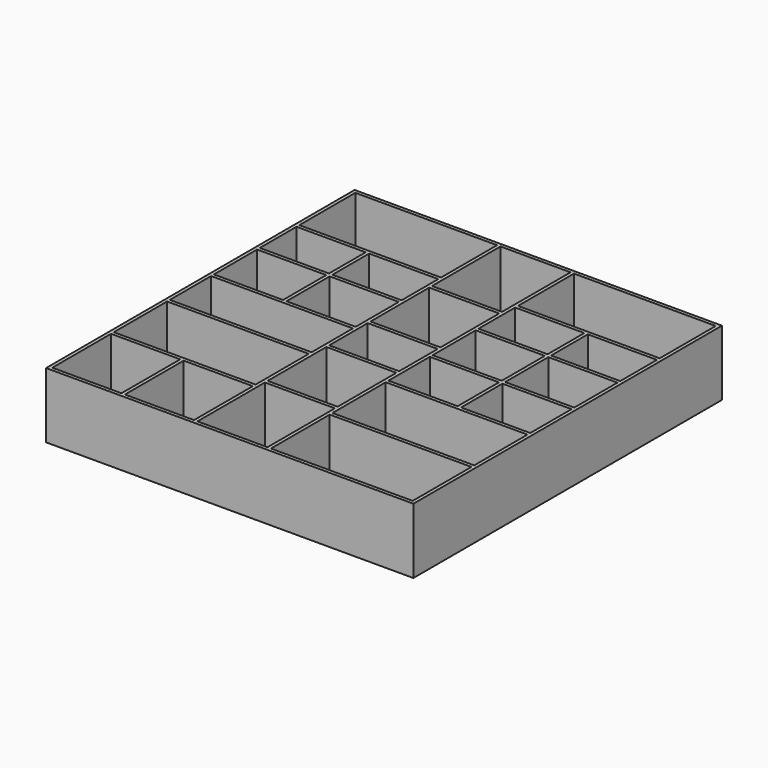
from build123d import *

# Parameters (mm, degrees)
F0_W     = 784.225
F0_H     = 387.35
F0_W_2   = 382.5875
F0_H_2   = 406.4
F0_H_3   = 254
F0_W_3   = 387.35
F0_H_4   = 473.7870542765
F0_W_4   = 19.05
F0_H_5   = 19.05
F0_H_6   = 368.3
F0_H_7   = 298.45
F0_H_8   = 466.0129457235
F0_H_9   = 285.75
F0_H_10  = 266.7
F1_DEPTH = 6.35
F2_DEPTH = 355.6


with BuildPart() as f1:
    # F0 (on Top) → F1 (new body)
    with BuildSketch(Plane.XY):
        Polygon((-1882.2203393722, 1059.8308014154), (-1901.2703393722, 1059.8308014154), (-1901.2703393722, -1073.7691985846), (-1882.2203393722, -1073.7691985846), (-1882.2203393722, -1054.7191985846), (-1882.2203393722, -648.3191985846), (-1882.2203393722, -629.2691985846), (-1882.2203393722, -260.9691985846), (-1882.2203393722, -241.9191985846), (-1882.2203393722, 43.8308014154), (-1882.2203393722, 62.8808014154), (-1882.2203393722, 361.3308014154), (-1882.2203393722, 380.3808014154), (-1882.2203393722, 634.3808014154), (-1882.2203393722, 653.4308014154), (-1882.2203393722, 1040.7808014154), align=None)
        Polygon((-682.0703393722, 1059.8308014154), (-1882.2203393722, 1059.8308014154), (-1882.2203393722, 1040.7808014154), (-1097.9953393722, 1040.7808014154), (-1078.9453393722, 1040.7808014154), (-691.5953393722, 1040.7808014154), (-672.5453393722, 1040.7808014154), (111.6796606278, 1040.7808014154), (111.6796606278, 1059.8308014154), align=None)
        with Locations((-1490.1078393722, 847.1058014154)):
            Rectangle(F0_W, F0_H)
        Polygon((-1882.2203393722, -1054.7191985846), (-1882.2203393722, -1073.7691985846), (111.6796606278, -1073.7691985846), (111.6796606278, -1054.7191985846), (-672.5453393722, -1054.7191985846), (-691.5953393722, -1054.7191985846), (-1078.9453393722, -1054.7191985846), (-1097.9953393722, -1054.7191985846), (-1480.5828393722, -1054.7191985846), (-1499.6328393722, -1054.7191985846), align=None)
        Polygon((130.7296606278, 1059.8308014154), (111.6796606278, 1059.8308014154), (111.6796606278, 1040.7808014154), (111.6796606278, 653.4308014154), (111.6796606278, 634.3808014154), (111.6796606278, 380.3808014154), (111.6796606278, 361.3308014154), (111.6796606278, 62.8808014154), (111.6796606278, 43.8308014154), (111.6796606278, -241.9191985846), (111.6796606278, -260.9691985846), (111.6796606278, -629.2691985846), (111.6796606278, -648.3191985846), (111.6796606278, -1054.7191985846), (111.6796606278, -1073.7691985846), (130.7296606278, -1073.7691985846), align=None)
        Polygon((-1097.9953393722, 653.4308014154), (-1882.2203393722, 653.4308014154), (-1882.2203393722, 634.3808014154), (-1499.6328393722, 634.3808014154), (-1480.5828393722, 634.3808014154), (-1097.9953393722, 634.3808014154), align=None)
        Polygon((-1078.9453393722, 1040.7808014154), (-1097.9953393722, 1040.7808014154), (-1097.9953393722, 653.4308014154), (-1097.9953393722, 634.3808014154), (-1097.9953393722, 380.3808014154), (-1097.9953393722, 361.3308014154), (-1097.9953393722, 62.8808014154), (-1097.9953393722, 43.8308014154), (-1097.9953393722, -241.9191985846), (-1097.9953393722, -260.9691985846), (-1097.9953393722, -629.2691985846), (-1097.9953393722, -648.3191985846), (-1097.9953393722, -1054.7191985846), (-1078.9453393722, -1054.7191985846), (-1078.9453393722, -588.706252861), (-1078.9453393722, -569.656252861), (-1078.9453393722, -163.256252861), (-1078.9453393722, -144.206252861), (-1078.9453393722, 122.493747139), (-1078.9453393722, 141.543747139), (-1078.9453393722, 547.943747139), (-1078.9453393722, 566.993747139), align=None)
        with Locations((-1690.9265893722, -851.5191985846)):
            Rectangle(F0_W_2, F0_H_2)
        with Locations((-280.4328393722, 847.1058014154)):
            Rectangle(F0_W, F0_H)
        with Locations((-1690.9265893722, 507.3808014154)):
            Rectangle(F0_W_2, F0_H_3)
        with Locations((-885.2703393722, 803.8872742772)):
            Rectangle(F0_W_3, F0_H_4)
        with Locations((-280.4328393722, -851.5191985846)):
            Rectangle(F0_W, F0_H_2)
        Polygon((-1882.2203393722, -629.2691985846), (-1882.2203393722, -648.3191985846), (-1499.6328393722, -648.3191985846), (-1480.5828393722, -648.3191985846), (-1097.9953393722, -648.3191985846), (-1097.9953393722, -629.2691985846), align=None)
        with Locations((-1490.1078393722, -851.5191985846)):
            Rectangle(F0_W_4, F0_H_2)
        Polygon((111.6796606278, 634.3808014154), (111.6796606278, 653.4308014154), (-672.5453393722, 653.4308014154), (-672.5453393722, 634.3808014154), (-289.9578393722, 634.3808014154), (-270.9078393722, 634.3808014154), align=None)
        Polygon((-672.5453393722, 653.4308014154), (-672.5453393722, 1040.7808014154), (-691.5953393722, 1040.7808014154), (-691.5953393722, 566.993747139), (-691.5953393722, 547.943747139), (-691.5953393722, 141.543747139), (-691.5953393722, 122.493747139), (-691.5953393722, -144.206252861), (-691.5953393722, -163.256252861), (-691.5953393722, -569.656252861), (-691.5953393722, -588.706252861), (-691.5953393722, -1054.7191985846), (-672.5453393722, -1054.7191985846), (-672.5453393722, -648.3191985846), (-672.5453393722, -629.2691985846), (-672.5453393722, -260.9691985846), (-672.5453393722, -241.9191985846), (-672.5453393722, 43.8308014154), (-672.5453393722, 62.8808014154), (-672.5453393722, 361.3308014154), (-672.5453393722, 380.3808014154), (-672.5453393722, 634.3808014154), align=None)
        with Locations((-1690.9265893722, 370.8558014154)):
            Rectangle(F0_W_2, F0_H_5)
        with Locations((-1490.1078393722, 507.3808014154)):
            Rectangle(F0_W_4, F0_H_3)
        with Locations((-1289.2890893722, 507.3808014154)):
            Rectangle(F0_W_2, F0_H_3)
        with Locations((-885.2703393722, 557.468747139)):
            Rectangle(F0_W_3, F0_H_5)
        with Locations((-280.4328393722, -638.7941985846)):
            Rectangle(F0_W, F0_H_5)
        with Locations((-1490.1078393722, -445.1191985846)):
            Rectangle(F0_W, F0_H_6)
        with Locations((-1289.2890893722, -851.5191985846)):
            Rectangle(F0_W_2, F0_H_2)
        with Locations((-79.6140893722, 507.3808014154)):
            Rectangle(F0_W_2, F0_H_3)
        with Locations((-1690.9265893722, 212.1058014154)):
            Rectangle(F0_W_2, F0_H_7)
        with Locations((-1490.1078393722, 370.8558014154)):
            Rectangle(F0_W_4, F0_H_5)
        with Locations((-1289.2890893722, 370.8558014154)):
            Rectangle(F0_W_2, F0_H_5)
        with Locations((-885.2703393722, 344.743747139)):
            Rectangle(F0_W_3, F0_H_2)
        with Locations((-280.4328393722, -445.1191985846)):
            Rectangle(F0_W, F0_H_6)
        with Locations((-885.2703393722, -821.7127257228)):
            Rectangle(F0_W_3, F0_H_8)
        with Locations((-1490.1078393722, -251.4441985846)):
            Rectangle(F0_W, F0_H_5)
        with Locations((-79.6140893722, 370.8558014154)):
            Rectangle(F0_W_2, F0_H_5)
        with Locations((-280.4328393722, 507.3808014154)):
            Rectangle(F0_W_4, F0_H_3)
        with Locations((-481.2515893722, 507.3808014154)):
            Rectangle(F0_W_2, F0_H_3)
        Polygon((-1499.6328393722, 62.8808014154), (-1882.2203393722, 62.8808014154), (-1882.2203393722, 43.8308014154), (-1097.9953393722, 43.8308014154), (-1097.9953393722, 62.8808014154), (-1480.5828393722, 62.8808014154), align=None)
        with Locations((-1490.1078393722, 212.1058014154)):
            Rectangle(F0_W_4, F0_H_7)
        with Locations((-1289.2890893722, 212.1058014154)):
            Rectangle(F0_W_2, F0_H_7)
        with Locations((-885.2703393722, 132.018747139)):
            Rectangle(F0_W_3, F0_H_5)
        Polygon((-672.5453393722, -260.9691985846), (111.6796606278, -260.9691985846), (111.6796606278, -241.9191985846), (-270.9078393722, -241.9191985846), (-289.9578393722, -241.9191985846), (-672.5453393722, -241.9191985846), align=None)
        with Locations((-885.2703393722, -579.181252861)):
            Rectangle(F0_W_3, F0_H_5)
        with Locations((-1490.1078393722, -99.0441985846)):
            Rectangle(F0_W, F0_H_9)
        with Locations((-79.6140893722, 212.1058014154)):
            Rectangle(F0_W_2, F0_H_7)
        with Locations((-280.4328393722, 370.8558014154)):
            Rectangle(F0_W_4, F0_H_5)
        with Locations((-481.2515893722, 370.8558014154)):
            Rectangle(F0_W_2, F0_H_5)
        with Locations((-885.2703393722, -10.856252861)):
            Rectangle(F0_W_3, F0_H_10)
        with Locations((-79.6140893722, -99.0441985846)):
            Rectangle(F0_W_2, F0_H_9)
        with Locations((-885.2703393722, -366.456252861)):
            Rectangle(F0_W_3, F0_H_2)
        with Locations((-79.6140893722, 53.3558014154)):
            Rectangle(F0_W_2, F0_H_5)
        with Locations((-280.4328393722, 212.1058014154)):
            Rectangle(F0_W_4, F0_H_7)
        with Locations((-481.2515893722, 212.1058014154)):
            Rectangle(F0_W_2, F0_H_7)
        with Locations((-885.2703393722, -153.731252861)):
            Rectangle(F0_W_3, F0_H_5)
        with Locations((-280.4328393722, -99.0441985846)):
            Rectangle(F0_W_4, F0_H_9)
        with Locations((-481.2515893722, -99.0441985846)):
            Rectangle(F0_W_2, F0_H_9)
        with Locations((-280.4328393722, 53.3558014154)):
            Rectangle(F0_W_4, F0_H_5)
        with Locations((-481.2515893722, 53.3558014154)):
            Rectangle(F0_W_2, F0_H_5)
    extrude(amount=-F1_DEPTH)

    # F0 (on Top) → F2 (join)
    with BuildSketch(Plane.XY):
        Polygon((-1882.2203393722, 1059.8308014154), (-1901.2703393722, 1059.8308014154), (-1901.2703393722, -1073.7691985846), (-1882.2203393722, -1073.7691985846), (-1882.2203393722, -1054.7191985846), (-1882.2203393722, -648.3191985846), (-1882.2203393722, -629.2691985846), (-1882.2203393722, -260.9691985846), (-1882.2203393722, -241.9191985846), (-1882.2203393722, 43.8308014154), (-1882.2203393722, 62.8808014154), (-1882.2203393722, 361.3308014154), (-1882.2203393722, 380.3808014154), (-1882.2203393722, 634.3808014154), (-1882.2203393722, 653.4308014154), (-1882.2203393722, 1040.7808014154), align=None)
        Polygon((-682.0703393722, 1059.8308014154), (-1882.2203393722, 1059.8308014154), (-1882.2203393722, 1040.7808014154), (-1097.9953393722, 1040.7808014154), (-1078.9453393722, 1040.7808014154), (-691.5953393722, 1040.7808014154), (-672.5453393722, 1040.7808014154), (111.6796606278, 1040.7808014154), (111.6796606278, 1059.8308014154), align=None)
        Polygon((-1882.2203393722, -1054.7191985846), (-1882.2203393722, -1073.7691985846), (111.6796606278, -1073.7691985846), (111.6796606278, -1054.7191985846), (-672.5453393722, -1054.7191985846), (-691.5953393722, -1054.7191985846), (-1078.9453393722, -1054.7191985846), (-1097.9953393722, -1054.7191985846), (-1480.5828393722, -1054.7191985846), (-1499.6328393722, -1054.7191985846), align=None)
        Polygon((130.7296606278, 1059.8308014154), (111.6796606278, 1059.8308014154), (111.6796606278, 1040.7808014154), (111.6796606278, 653.4308014154), (111.6796606278, 634.3808014154), (111.6796606278, 380.3808014154), (111.6796606278, 361.3308014154), (111.6796606278, 62.8808014154), (111.6796606278, 43.8308014154), (111.6796606278, -241.9191985846), (111.6796606278, -260.9691985846), (111.6796606278, -629.2691985846), (111.6796606278, -648.3191985846), (111.6796606278, -1054.7191985846), (111.6796606278, -1073.7691985846), (130.7296606278, -1073.7691985846), align=None)
        Polygon((-1097.9953393722, 653.4308014154), (-1882.2203393722, 653.4308014154), (-1882.2203393722, 634.3808014154), (-1499.6328393722, 634.3808014154), (-1480.5828393722, 634.3808014154), (-1097.9953393722, 634.3808014154), align=None)
        Polygon((-1078.9453393722, 1040.7808014154), (-1097.9953393722, 1040.7808014154), (-1097.9953393722, 653.4308014154), (-1097.9953393722, 634.3808014154), (-1097.9953393722, 380.3808014154), (-1097.9953393722, 361.3308014154), (-1097.9953393722, 62.8808014154), (-1097.9953393722, 43.8308014154), (-1097.9953393722, -241.9191985846), (-1097.9953393722, -260.9691985846), (-1097.9953393722, -629.2691985846), (-1097.9953393722, -648.3191985846), (-1097.9953393722, -1054.7191985846), (-1078.9453393722, -1054.7191985846), (-1078.9453393722, -588.706252861), (-1078.9453393722, -569.656252861), (-1078.9453393722, -163.256252861), (-1078.9453393722, -144.206252861), (-1078.9453393722, 122.493747139), (-1078.9453393722, 141.543747139), (-1078.9453393722, 547.943747139), (-1078.9453393722, 566.993747139), align=None)
        Polygon((-1882.2203393722, -629.2691985846), (-1882.2203393722, -648.3191985846), (-1499.6328393722, -648.3191985846), (-1480.5828393722, -648.3191985846), (-1097.9953393722, -648.3191985846), (-1097.9953393722, -629.2691985846), align=None)
        with Locations((-1490.1078393722, -851.5191985846)):
            Rectangle(F0_W_4, F0_H_2)
        Polygon((111.6796606278, 634.3808014154), (111.6796606278, 653.4308014154), (-672.5453393722, 653.4308014154), (-672.5453393722, 634.3808014154), (-289.9578393722, 634.3808014154), (-270.9078393722, 634.3808014154), align=None)
        Polygon((-672.5453393722, 653.4308014154), (-672.5453393722, 1040.7808014154), (-691.5953393722, 1040.7808014154), (-691.5953393722, 566.993747139), (-691.5953393722, 547.943747139), (-691.5953393722, 141.543747139), (-691.5953393722, 122.493747139), (-691.5953393722, -144.206252861), (-691.5953393722, -163.256252861), (-691.5953393722, -569.656252861), (-691.5953393722, -588.706252861), (-691.5953393722, -1054.7191985846), (-672.5453393722, -1054.7191985846), (-672.5453393722, -648.3191985846), (-672.5453393722, -629.2691985846), (-672.5453393722, -260.9691985846), (-672.5453393722, -241.9191985846), (-672.5453393722, 43.8308014154), (-672.5453393722, 62.8808014154), (-672.5453393722, 361.3308014154), (-672.5453393722, 380.3808014154), (-672.5453393722, 634.3808014154), align=None)
        with Locations((-1690.9265893722, 370.8558014154)):
            Rectangle(F0_W_2, F0_H_5)
        with Locations((-1490.1078393722, 507.3808014154)):
            Rectangle(F0_W_4, F0_H_3)
        with Locations((-885.2703393722, 557.468747139)):
            Rectangle(F0_W_3, F0_H_5)
        with Locations((-280.4328393722, -638.7941985846)):
            Rectangle(F0_W, F0_H_5)
        with Locations((-1490.1078393722, 370.8558014154)):
            Rectangle(F0_W_4, F0_H_5)
        with Locations((-1289.2890893722, 370.8558014154)):
            Rectangle(F0_W_2, F0_H_5)
        with Locations((-1490.1078393722, -251.4441985846)):
            Rectangle(F0_W, F0_H_5)
        with Locations((-79.6140893722, 370.8558014154)):
            Rectangle(F0_W_2, F0_H_5)
        with Locations((-280.4328393722, 507.3808014154)):
            Rectangle(F0_W_4, F0_H_3)
        Polygon((-1499.6328393722, 62.8808014154), (-1882.2203393722, 62.8808014154), (-1882.2203393722, 43.8308014154), (-1097.9953393722, 43.8308014154), (-1097.9953393722, 62.8808014154), (-1480.5828393722, 62.8808014154), align=None)
        with Locations((-1490.1078393722, 212.1058014154)):
            Rectangle(F0_W_4, F0_H_7)
        with Locations((-885.2703393722, 132.018747139)):
            Rectangle(F0_W_3, F0_H_5)
        Polygon((-672.5453393722, -260.9691985846), (111.6796606278, -260.9691985846), (111.6796606278, -241.9191985846), (-270.9078393722, -241.9191985846), (-289.9578393722, -241.9191985846), (-672.5453393722, -241.9191985846), align=None)
        with Locations((-885.2703393722, -579.181252861)):
            Rectangle(F0_W_3, F0_H_5)
        with Locations((-280.4328393722, 370.8558014154)):
            Rectangle(F0_W_4, F0_H_5)
        with Locations((-481.2515893722, 370.8558014154)):
            Rectangle(F0_W_2, F0_H_5)
        with Locations((-79.6140893722, 53.3558014154)):
            Rectangle(F0_W_2, F0_H_5)
        with Locations((-280.4328393722, 212.1058014154)):
            Rectangle(F0_W_4, F0_H_7)
        with Locations((-885.2703393722, -153.731252861)):
            Rectangle(F0_W_3, F0_H_5)
        with Locations((-280.4328393722, -99.0441985846)):
            Rectangle(F0_W_4, F0_H_9)
        with Locations((-280.4328393722, 53.3558014154)):
            Rectangle(F0_W_4, F0_H_5)
        with Locations((-481.2515893722, 53.3558014154)):
            Rectangle(F0_W_2, F0_H_5)
    extrude(amount=F2_DEPTH)


solid = f1.part
